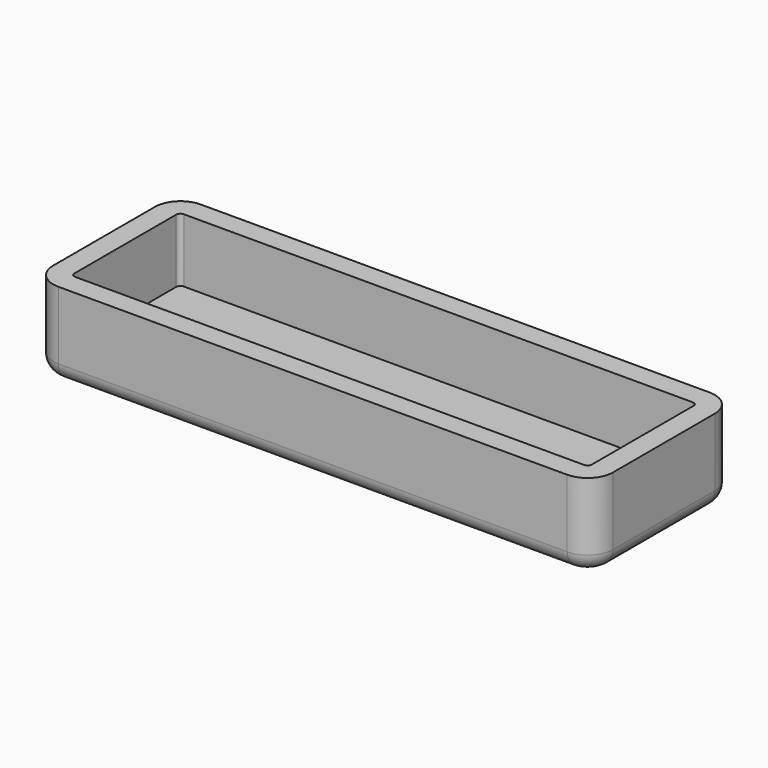
from build123d import *

# Parameters (mm, degrees)
F1_DEPTH = 10
F2_T     = -2.5
F3_R     = 1.9452355594
F4_DEPTH = 2.501
F6_R     = 2


# Not quite as in the source:
# - a fillet or chamfer that OpenCascade refuses, or shapes differently, is made with other operations: its cross-section is extruded or revolved along the edge and cut away or added


with BuildPart() as f1:
    # F0 (on Top) → F1 (new body)
    with BuildSketch(Plane.XY):
        with BuildLine():
            Line((-30, -10.5), (30, -10.5))
            ThreePointArc((30, -10.5), (32.1213203436, -9.6213203436), (33, -7.5))
            Line((33, -7.5), (33, 7.5))
            ThreePointArc((33, 7.5), (32.1213203436, 9.6213203436), (30, 10.5))
            Line((30, 10.5), (-30, 10.5))
            ThreePointArc((-30, 10.5), (-32.1213203436, 9.6213203436), (-33, 7.5))
            Line((-33, 7.5), (-33, -7.5))
            ThreePointArc((-33, -7.5), (-32.1213203436, -9.6213203436), (-30, -10.5))
        make_face()
    extrude(amount=F1_DEPTH)

    # F2
    f2_openings = [f1.faces().sort_by_distance(p)[0] for p in [
        (0, 0, 10),
    ]]
    offset(amount=F2_T, openings=f2_openings)

    # F3 (on face) → F4 (cut, through all)
    with BuildSketch(Plane.XY.offset(2.5)):
        with Locations((-23.9163879305, 0)):
            Circle(F3_R)
        with Locations((23.9163879305, 0)):
            Circle(F3_R)
    extrude(amount=-F4_DEPTH, mode=Mode.SUBTRACT)

    # F5: chamfer of 3 on 2 edges, made by hand

    # F5_s1 → F5_t2 (revolve, cut)
    with BuildSketch(Plane.XZ):
        Polygon((28.8616234899, 0), (25.8616234899, 3), (25.8616234899, 0), align=None)
    revolve(axis=Axis((23.9163879305, 0, 0), (0, 0, 1)), mode=Mode.SUBTRACT)

    # F5_s3 → F5_t4 (revolve, cut)
    with BuildSketch(Plane.XZ):
        Polygon((-18.9711523711, 0), (-21.9711523711, 3), (-21.9711523711, 0), align=None)
    revolve(axis=Axis((-23.9163879305, 0, 0), (0, 0, 1)), mode=Mode.SUBTRACT)

    # F6
    f6_edges = [f1.edges().sort_by_distance(p)[0] for p in [
        (0, -10.5, 0),
        (-32.12132, -9.62132, 0),
        (32.12132, -9.62132, 0),
        (-33, 0, 0),
        (33, 0, 0),
        (-32.12132, 9.62132, 0),
        (32.12132, 9.62132, 0),
        (0, 10.5, 0),
        (-28.861623, 0, 0),
        (18.971152, 0, 0),
    ]]
    fillet(f6_edges, radius=F6_R)


solid = f1.part
